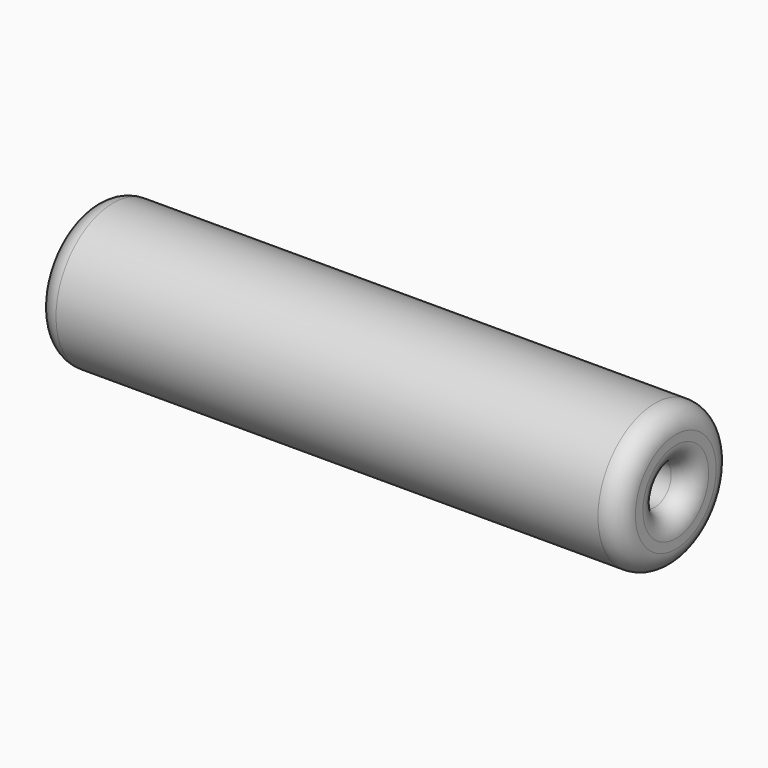
from build123d import *

# Parameters (mm, degrees)
F1_W = 140.3701454401
F1_H = 12.250483036
F5_R = 5
F6_R = 5


# Not quite as in the source:
# - a feature of the source that left no trace in its solid (it failed there, or was rolled back) is left out


with BuildPart() as f4:
    # F1 (on Front) → F4 (revolve)
    with BuildSketch(Plane.XZ):
        with Locations((270.1073512435, 393.0281996727)):
            Rectangle(F1_W, F1_H)
    revolve(axis=Axis((279.5873135328, 0, 382.010191679), (1, 0, 0)))

    # F5
    f5_edges = [f4.edges().sort_by_distance(p)[0] for p in [
        (340.292424, 0, 377.117425),
        (340.292424, 0, 364.866942),
    ]]
    fillet(f5_edges, radius=F5_R)

    # F6
    f6_edges = [f4.edges().sort_by_distance(p)[0] for p in [
        (199.922279, 0, 364.866942),
        (199.922279, 0, 377.117425),
    ]]
    fillet(f6_edges, radius=F6_R)


solid = f4.part
